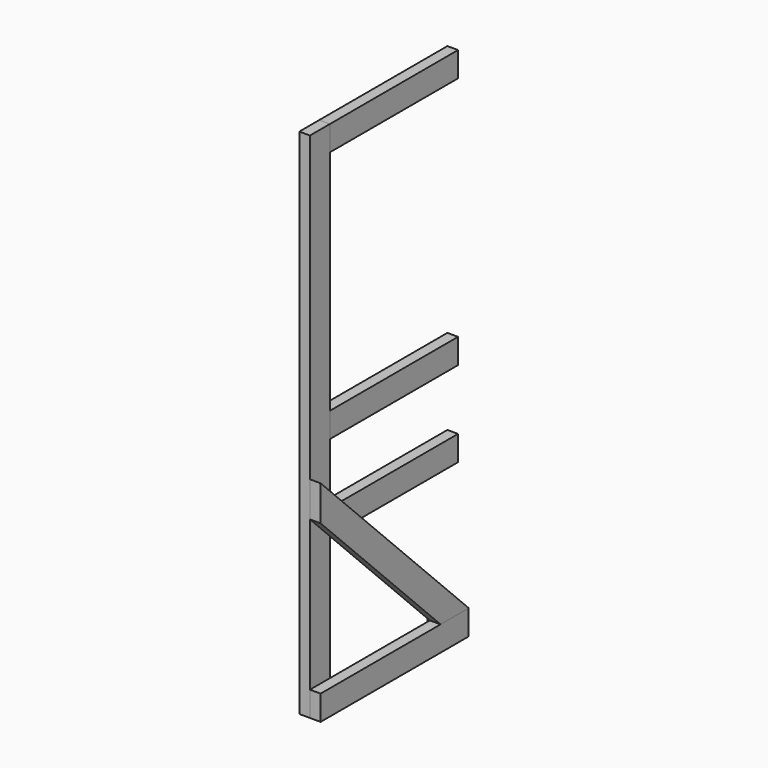
from build123d import *

# Parameters (mm, degrees)
F0_W     = 660.4
F0_H     = 88.9
F1_DEPTH = 38.1
F2_W     = 88.9
F2_H     = 1828.8
F3_DEPTH = 38.1
F5_DEPTH = 38.1
F7_DEPTH = 38.1
F8_W     = 571.5
F8_H     = 88.9
F9_DEPTH = 38.1


with BuildPart() as f1:
    # F0 (on Right) → F1 (new body)
    with BuildSketch(Plane.YZ):
        with Locations((330.2, 44.45)):
            Rectangle(F0_W, F0_H)
    extrude(amount=F1_DEPTH)


with BuildPart() as f3:
    # F2 (on Right) → F3 (new body)
    with BuildSketch(Plane.YZ):
        with Locations((44.45, 914.4)):
            Rectangle(F2_W, F2_H)
    extrude(amount=-F3_DEPTH)


with BuildPart() as f5:
    # F4 (on Right) → F5 (new body)
    with BuildSketch(Plane.YZ):
        Polygon((660.4, 88.9), (0, 749.3), (0, 623.576414305), (534.676414305, 88.9), align=None)
    extrude(amount=F5_DEPTH)


with BuildPart() as f7:
    # F6 (on face) → F7 (new body)
    with BuildSketch(Plane(origin=(0, 0, 0), x_dir=(0, -1, 0), z_dir=(-1, 0, 0))):
        Polygon((-660.4, 88.9), (-660.4, 0), (-571.5, 0), (-571.5, 177.8), align=None)
    extrude(amount=F7_DEPTH)


with BuildPart() as f9:
    # F8 (on face) → F9 (new body)
    with BuildSketch(Plane(origin=(0, 0, 0), x_dir=(0, -1, 0), z_dir=(-1, 0, 0))):
        with Locations((-374.65, 579.126414305)):
            Rectangle(F8_W, F8_H)
    extrude(amount=F9_DEPTH)


with BuildPart() as f10_1:
    # F10: copy of F9
    add(f9.part.moved(Location((0, 0, 304.8))))


with BuildPart() as f13_1:
    # F13: copy of F9
    add(f9.part.moved(Location((0, 0, 1205.223585695))))


solid = Compound([f1.part, f3.part, f5.part, f7.part, f9.part, f10_1.part, f13_1.part])
